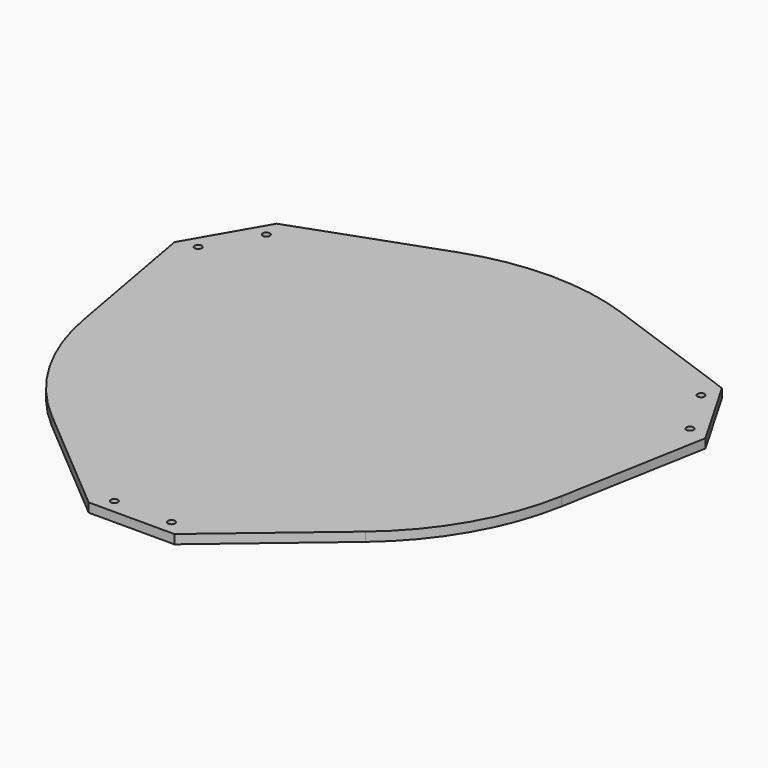
from build123d import *

# Parameters (mm, degrees)
F0_R     = 2.5
F1_DEPTH = 6.35


# Not quite as in the source:
# - a length typed as a fraction of an inch, garbled in the dataset ("3 / 203.2 mm" for 3/8 in), is restored


with BuildPart() as f1:
    # F0 (on Top) → F1 (new body)
    with BuildSketch(Plane.XY):
        with BuildLine():
            Line((-79.8226374756, -129.7651274337), (0, -197.3205080757))
            Line((0, -197.3205080757), (60, -197.3205080757))
            Line((60, -197.3205080757), (139.8226374756, -129.7651274337))
            ThreePointArc((139.8226374756, -129.7651274337), (177.2243186434, -85), (197.2912156208, -30.2266302477))
            Line((197.2912156208, -30.2266302477), (215.8845726812, 72.6794919243))
            Line((215.8845726812, 72.6794919243), (185.8845726812, 124.6410161514))
            Line((185.8845726812, 124.6410161514), (87.4685781451, 159.9917576814))
            ThreePointArc((87.4685781451, 159.9917576814), (30, 170), (-27.4685781451, 159.9917576814))
            Line((-27.4685781451, 159.9917576814), (-125.8845726812, 124.6410161514))
            Line((-125.8845726812, 124.6410161514), (-155.8845726812, 72.6794919243))
            Line((-155.8845726812, 72.6794919243), (-137.2912156208, -30.2266302477))
            ThreePointArc((-137.2912156208, -30.2266302477), (-117.2243186434, -85), (-79.8226374756, -129.7651274337))
        make_face()
        with Locations((10, -187.3205080757)):
            Circle(F0_R, mode=Mode.SUBTRACT)
        with Locations((50, -187.3205080757)):
            Circle(F0_R, mode=Mode.SUBTRACT)
        with Locations((-142.2243186434, 76.3397459622)):
            Circle(F0_R, mode=Mode.SUBTRACT)
        with Locations((-122.2243186434, 110.9807621135)):
            Circle(F0_R, mode=Mode.SUBTRACT)
        with Locations((202.2243186434, 76.3397459622)):
            Circle(F0_R, mode=Mode.SUBTRACT)
        with Locations((182.2243186434, 110.9807621135)):
            Circle(F0_R, mode=Mode.SUBTRACT)
    extrude(amount=F1_DEPTH)


solid = f1.part
